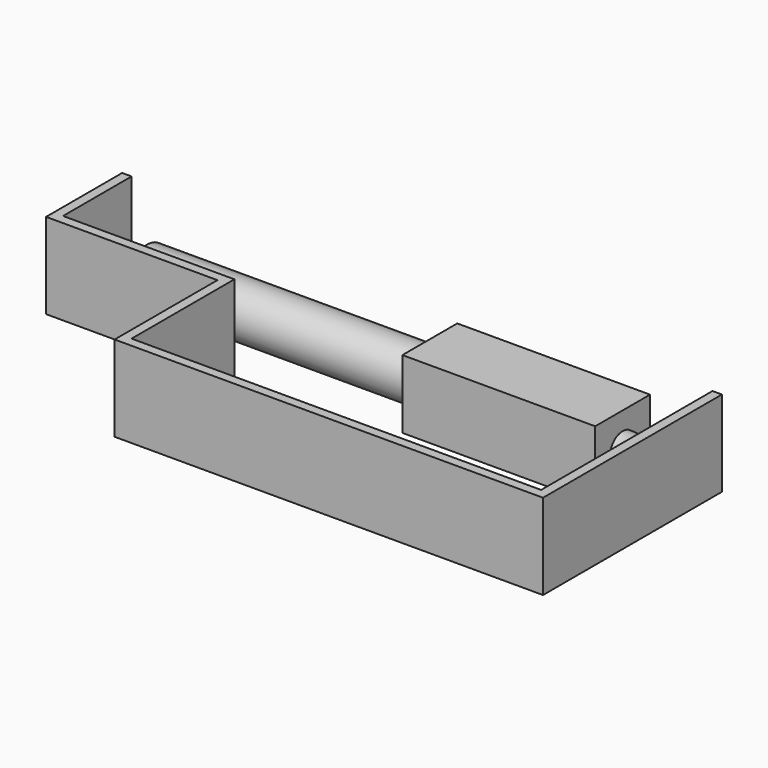
from build123d import *

# Parameters (mm, degrees)
F0_W     = 450
F0_H     = 160
F1_DEPTH = 160
F3_DEPTH = 200
F4_R     = 60
F5_DEPTH = 660
F6_R     = 37.5
F9_DEPTH = 317.7312946493


with BuildPart() as f1:
    # F0 (on Top) → F1 (new body)
    with BuildSketch(Plane.XY):
        with Locations((-375, -102.2687053507)):
            Rectangle(F0_W, F0_H)
    extrude(amount=F1_DEPTH)

    # F4 (on face) → F5 (join)
    with BuildSketch(Plane(origin=(-600, 0, 0), x_dir=(0, -1, 0), z_dir=(-1, 0, 0))):
        with Locations((102.2687053507, 80)):
            Circle(F4_R)
    extrude(amount=F5_DEPTH)

    # F8: sweep along a path in F7
    with BuildLine(Plane.XY) as f8_path:
        ThreePointArc((-70, -182.2687053507), (-93.4314575051, -125.7001628558), (-150, -102.2687053507))
    # F6 (on face) → F8 (sweep)
    with BuildSketch(Plane.YZ.offset(-150)):
        with Locations((-102.2687053507, 80)):
            Circle(F6_R)
    sweep(path=f8_path.line)

    # F9 (add, through all): a face of the model
    f9_faces = [f1.faces().sort_by_distance(p)[0] for p in [
        (-70, -182.2687053507, 80),
    ]]
    extrude(f9_faces, amount=F9_DEPTH)


with BuildPart() as f3:
    # F2 (on Top) → F3 (new body)
    with BuildSketch(Plane.XY):
        Polygon((0, -522), (0, 0), (-22, 0), (-22, -500), (-978, -500), (-978, -200), (-1378, -200), (-1378, 0), (-1400, 0), (-1400, -222), (-1000, -222), (-1000, -522), align=None)
    extrude(amount=F3_DEPTH)


solid = Compound([f1.part, f3.part])
